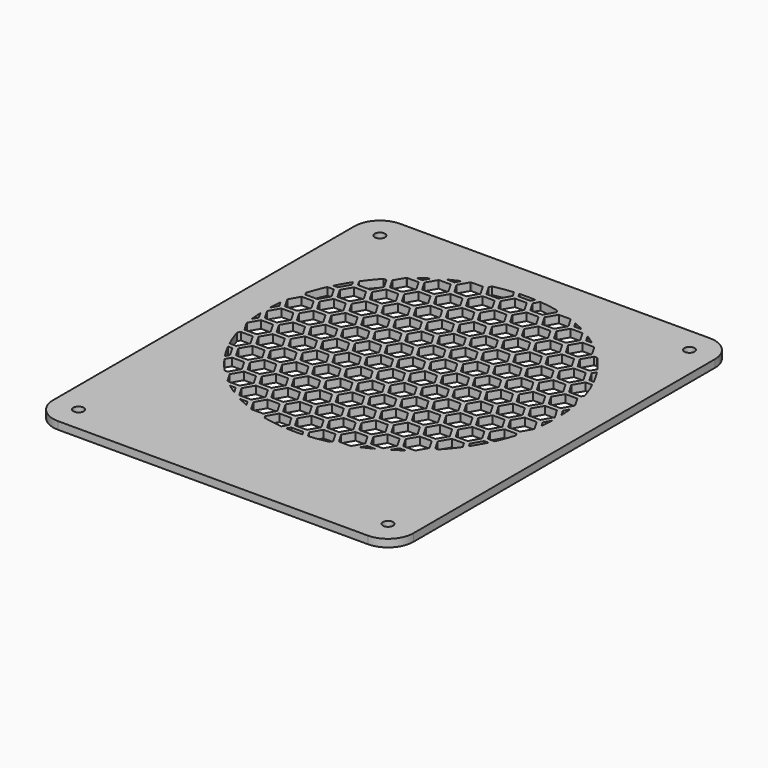
from build123d import *

# Parameters (mm, degrees)
F0_R     = 2
F0_R_2   = 4.5
F1_DEPTH = 3
F2_DEPTH = 2


# Not quite as in the source:
# - ends of sketch curves that miss each other by under 0.0002 mm in the source are joined


with BuildPart() as f1:
    # F0 (on Top) → F1 (new body)
    with BuildSketch(Plane.XY):
        with BuildLine():
            Line((61, 71), (-61, 71))
            ThreePointArc((-61, 71), (-68.0710678119, 68.0710678119), (-71, 61))
            Line((-71, 61), (-71, -87.5))
            ThreePointArc((-71, -87.5), (-68.0710678119, -94.5710678119), (-61, -97.5))
            Line((-61, -97.5), (61, -97.5))
            ThreePointArc((61, -97.5), (68.0710678119, -94.5710678119), (71, -87.5))
            Line((71, -87.5), (71, 61))
            ThreePointArc((71, 61), (68.0710678119, 68.0710678119), (61, 71))
        make_face()
        with Locations((-61, -87.5)):
            Circle(F0_R, mode=Mode.SUBTRACT)
        with Locations((-52.2617718254, -52.3417506076)):
            Circle(F0_R_2, mode=Mode.SUBTRACT)
        with BuildLine():
            Line((-45.6730132859, -30.9579411415), (-40.9387409983, -30.9579411415))
            Line((-40.9387409983, -30.9579411415), (-38.5716048624, -35.0579411973))
            Line((-38.5716048624, -35.0579411973), (-40.9387411583, -39.1579412804))
            Line((-40.9387411583, -39.1579412804), (-42.1058859861, -39.1579412804))
            ThreePointArc((-42.1058859861, -39.1579412804), (-44.6321134172, -36.2522337507), (-46.9582140117, -33.1839740965))
            Line((-46.9582140117, -33.1839740965), (-45.6730132859, -30.9579411415))
        make_face(mode=Mode.SUBTRACT)
        with BuildLine():
            Line((-49.5989950362, -25.9579412533), (-47.2318589003, -30.057941309))
            Line((-47.2318589003, -30.057941309), (-48.0829899864, -31.5321435042))
            ThreePointArc((-48.0829899864, -31.5321435042), (-49.7732212515, -28.7902144182), (-51.3072634808, -25.9579412533))
            Line((-51.3072634808, -25.9579412533), (-49.5989950362, -25.9579412533))
        make_face(mode=Mode.SUBTRACT)
        Polygon((-40.9387409983, -20.8999998188), (-38.5716048624, -24.9999998745), (-40.9387411583, -29.0999999577), (-45.6730132859, -29.0999999577), (-48.0401494297, -24.9999998882), (-45.6730132859, -20.8999998188), align=None, mode=Mode.SUBTRACT)
        with BuildLine():
            Line((-49.5989950362, -15.8999999305), (-47.2318589003, -19.9999999863))
            Line((-47.2318589003, -19.9999999863), (-49.5989951961, -24.1000000695))
            Line((-49.5989951961, -24.1000000695), (-52.205746778, -24.1000000695))
            ThreePointArc((-52.205746778, -24.1000000695), (-53.6933380954, -20.5736589885), (-54.9430464582, -16.9561683729))
            Line((-54.9430464582, -16.9561683729), (-54.3332673237, -15.8999999305))
            Line((-54.3332673237, -15.8999999305), (-49.5989950362, -15.8999999305))
        make_face(mode=Mode.SUBTRACT)
        Polygon((-45.6730132859, -19.0999999577), (-48.0401494297, -14.9999998882), (-45.6730132859, -10.8999998188), (-40.9387409983, -10.8999998188), (-38.5716048624, -14.9999998745), (-40.9387411583, -19.0999999577), align=None, mode=Mode.SUBTRACT)
        with BuildLine():
            Line((-34.5560072312, -45.9579412533), (-32.2738800076, -45.9579412533))
            Line((-32.2738800076, -45.9579412533), (-30.7595285917, -48.5808748462))
            ThreePointArc((-30.7595285917, -48.5808748462), (-32.6840901681, -47.3075073311), (-34.5560072312, -45.9579412533))
        make_face(mode=Mode.SUBTRACT)
        with BuildLine():
            Line((-26.6371586929, -50.9579412533), (-23.6136263521, -50.9579412533))
            Line((-23.6136263521, -50.9579412533), (-22.4784041459, -52.9242037923))
            ThreePointArc((-22.4784041459, -52.9242037923), (-24.5774525803, -51.9826781213), (-26.6371586929, -50.9579412533))
        make_face(mode=Mode.SUBTRACT)
        Polygon((-23.6136263521, -40.9579412533), (-21.2464902162, -45.057941309), (-23.6136265121, -49.1579413922), (-28.3478986397, -49.1579413922), (-30.7150347835, -45.0579413227), (-28.3478986397, -40.9579412533), align=None, mode=Mode.SUBTRACT)
        with BuildLine():
            Line((-39.3752884389, -40.0579413227), (-37.0081522952, -35.9579412533))
            Line((-37.0081522952, -35.9579412533), (-32.2738800076, -35.9579412533))
            Line((-32.2738800076, -35.9579412533), (-29.9067438717, -40.057941309))
            Line((-29.9067438717, -40.057941309), (-32.2738801675, -44.1579413922))
            Line((-32.2738801675, -44.1579413922), (-36.8283343637, -44.1579413922))
            ThreePointArc((-36.8283343637, -44.1579413922), (-37.0033480808, -44.0113875129), (-37.1777786102, -43.8641399963))
            Line((-37.1777786102, -43.8641399963), (-39.3752884389, -40.0579413227))
        make_face(mode=Mode.SUBTRACT)
        Polygon((-30.7150347835, -35.0579413227), (-28.3478986397, -30.9579412533), (-23.6136263521, -30.9579412533), (-21.2464902162, -35.057941309), (-23.6136265121, -39.1579413922), (-28.3478986397, -39.1579413922), align=None, mode=Mode.SUBTRACT)
        with BuildLine():
            Line((-14.9533722834, -45.9579412533), (-12.5862361476, -50.057941309))
            Line((-12.5862361476, -50.057941309), (-14.9533724434, -54.1579413922))
            Line((-14.9533724434, -54.1579413922), (-19.3175408414, -54.1579413922))
            ThreePointArc((-19.3175408414, -54.1579413922), (-19.5515976014, -54.0738849283), (-19.7852886212, -53.9888169363))
            Line((-19.7852886212, -53.9888169363), (-22.0547807148, -50.0579413227))
            Line((-22.0547807148, -50.0579413227), (-19.687644571, -45.9579412533))
            Line((-19.687644571, -45.9579412533), (-14.9533722834, -45.9579412533))
        make_face(mode=Mode.SUBTRACT)
        with BuildLine():
            Line((-6.2931178941, -50.9579412533), (-3.9259817582, -55.057941309))
            Line((-3.9259817582, -55.057941309), (-5.199880045, -57.2643977312))
            ThreePointArc((-5.199880045, -57.2643977312), (-9.030429388, -56.7864538871), (-12.8202778486, -56.0525688607))
            Line((-12.8202778486, -56.0525688607), (-13.3945263254, -55.0579413227))
            Line((-13.3945263254, -55.0579413227), (-11.0273901816, -50.9579412533))
            Line((-11.0273901816, -50.9579412533), (-6.2931178941, -50.9579412533))
        make_face(mode=Mode.SUBTRACT)
        Polygon((-13.3945263254, -45.0579413227), (-11.0273901816, -40.9579412533), (-6.2931178941, -40.9579412533), (-3.9259817582, -45.057941309), (-6.293118054, -49.1579413922), (-11.0273901816, -49.1579413922), align=None, mode=Mode.SUBTRACT)
        Polygon((-19.687644571, -44.1579413922), (-22.0547807148, -40.0579413227), (-19.687644571, -35.9579412533), (-14.9533722834, -35.9579412533), (-12.5862361476, -40.057941309), (-14.9533724434, -44.1579413922), align=None, mode=Mode.SUBTRACT)
        Polygon((-13.3945263254, -35.0579413227), (-11.0273901816, -30.9579412533), (-6.2931178941, -30.9579412533), (-3.9259817582, -35.057941309), (-6.293118054, -39.1579413922), (-11.0273901816, -39.1579413922), align=None, mode=Mode.SUBTRACT)
        Polygon((-32.2738800076, -25.9579412533), (-29.9067438717, -30.057941309), (-32.2738801675, -34.1579413922), (-37.0081522952, -34.1579413922), (-39.3752884389, -30.0579413227), (-37.0081522952, -25.9579412533), align=None, mode=Mode.SUBTRACT)
        Polygon((-21.2464902162, -24.9999999863), (-23.6136265121, -29.1000000695), (-28.3478986397, -29.1000000695), (-30.7150347835, -25), (-28.3478986397, -20.8999999305), (-23.6136263521, -20.8999999305), align=None, mode=Mode.SUBTRACT)
        Polygon((-39.3752884389, -20), (-37.0081522952, -15.8999999305), (-32.2738800076, -15.8999999305), (-29.9067438717, -19.9999999863), (-32.2738801675, -24.1000000695), (-37.0081522952, -24.1000000695), align=None, mode=Mode.SUBTRACT)
        Polygon((-23.6136263521, -10.8999999305), (-21.2464902162, -14.9999999863), (-23.6136265121, -19.1000000695), (-28.3478986397, -19.1000000695), (-30.7150347835, -15), (-28.3478986397, -10.8999999305), align=None, mode=Mode.SUBTRACT)
        Polygon((-22.0547807148, -30.0579413227), (-19.687644571, -25.9579412533), (-14.9533722834, -25.9579412533), (-12.5862361476, -30.057941309), (-14.9533724434, -34.1579413922), (-19.687644571, -34.1579413922), align=None, mode=Mode.SUBTRACT)
        Polygon((-3.9259817582, -24.9999999863), (-6.293118054, -29.1000000695), (-11.0273901816, -29.1000000695), (-13.3945263254, -25), (-11.0273901816, -20.8999999305), (-6.2931178941, -20.8999999305), align=None, mode=Mode.SUBTRACT)
        Polygon((-14.9533722834, -15.8999999305), (-12.5862361476, -19.9999999863), (-14.9533724434, -24.1000000695), (-19.687644571, -24.1000000695), (-22.0547807148, -20), (-19.687644571, -15.8999999305), align=None, mode=Mode.SUBTRACT)
        Polygon((-3.9259817582, -14.9999999863), (-6.293118054, -19.1000000695), (-11.0273901816, -19.1000000695), (-13.3945263254, -15), (-11.0273901816, -10.8999999305), (-6.2931178941, -10.8999999305), align=None, mode=Mode.SUBTRACT)
        with BuildLine():
            Line((-2.3671363196, -55.9579410298), (0, -55.9579410298))
            Line((0, -55.9579410298), (2.3671363196, -55.9579410298))
            Line((2.3671363196, -55.9579410298), (3.2058082538, -57.4105634308))
            ThreePointArc((3.2058082538, -57.4105634308), (0, -57.5), (-3.2058082538, -57.4105634308))
            Line((-3.2058082538, -57.4105634308), (-2.3671363196, -55.9579410298))
        make_face(mode=Mode.SUBTRACT)
        with Locations((61, -87.5)):
            Circle(F0_R, mode=Mode.SUBTRACT)
        with BuildLine():
            Line((5.199880045, -57.2643977312), (3.9259817582, -55.057941309))
            Line((3.9259817582, -55.057941309), (6.2931178941, -50.9579412533))
            Line((6.2931178941, -50.9579412533), (11.0273901816, -50.9579412533))
            Line((11.0273901816, -50.9579412533), (13.3945263254, -55.0579413227))
            Line((13.3945263254, -55.0579413227), (12.8202778486, -56.0525688607))
            ThreePointArc((12.8202778486, -56.0525688607), (9.030429388, -56.7864538871), (5.199880045, -57.2643977312))
        make_face(mode=Mode.SUBTRACT)
        Polygon((-2.3671363196, -45.9579410298), (0, -45.9579410298), (2.3671363196, -45.9579410298), (4.7342724633, -50.0579410992), (2.3671363196, -54.1579411687), (0, -54.1579411687), (-2.3671363196, -54.1579411687), (-4.7342724633, -50.0579410992), align=None, mode=Mode.SUBTRACT)
        Polygon((11.0273901816, -40.9579412533), (13.3945263254, -45.0579413227), (11.0273901816, -49.1579413922), (6.293118054, -49.1579413922), (3.9259817582, -45.057941309), (6.2931178941, -40.9579412533), align=None, mode=Mode.SUBTRACT)
        with BuildLine():
            Line((19.3175408414, -54.1579413922), (14.9533724434, -54.1579413922))
            Line((14.9533724434, -54.1579413922), (12.5862361476, -50.057941309))
            Line((12.5862361476, -50.057941309), (14.9533722834, -45.9579412533))
            Line((14.9533722834, -45.9579412533), (19.687644571, -45.9579412533))
            Line((19.687644571, -45.9579412533), (22.0547807148, -50.0579413227))
            Line((22.0547807148, -50.0579413227), (19.7852886212, -53.9888169363))
            ThreePointArc((19.7852886212, -53.9888169363), (19.5515976014, -54.0738849283), (19.3175408414, -54.1579413922))
        make_face(mode=Mode.SUBTRACT)
        Polygon((2.3671363196, -44.1579411687), (0, -44.1579411687), (-2.3671363196, -44.1579411687), (-4.7342724633, -40.0579410992), (-2.3671363196, -35.9579410298), (0, -35.9579410298), (2.3671363196, -35.9579410298), (4.7342724633, -40.0579410992), align=None, mode=Mode.SUBTRACT)
        Polygon((11.0273901816, -30.9579412533), (13.3945263254, -35.0579413227), (11.0273901816, -39.1579413922), (6.293118054, -39.1579413922), (3.9259817582, -35.057941309), (6.2931178941, -30.9579412533), align=None, mode=Mode.SUBTRACT)
        Polygon((19.687644571, -44.1579413922), (14.9533724434, -44.1579413922), (12.5862361476, -40.057941309), (14.9533722834, -35.9579412533), (19.687644571, -35.9579412533), (22.0547807148, -40.0579413227), align=None, mode=Mode.SUBTRACT)
        with BuildLine():
            ThreePointArc((26.6371586929, -50.9579412533), (24.5774525803, -51.9826781213), (22.4784041459, -52.9242037923))
            Line((22.4784041459, -52.9242037923), (23.6136263521, -50.9579412533))
            Line((23.6136263521, -50.9579412533), (26.6371586929, -50.9579412533))
        make_face(mode=Mode.SUBTRACT)
        Polygon((28.3478986397, -40.9579412533), (30.7150347835, -45.0579413227), (28.3478986397, -49.1579413922), (23.6136265121, -49.1579413922), (21.2464902162, -45.057941309), (23.6136263521, -40.9579412533), align=None, mode=Mode.SUBTRACT)
        with BuildLine():
            ThreePointArc((34.5560072312, -45.9579412533), (32.6840901681, -47.3075073311), (30.7595285917, -48.5808748462))
            Line((30.7595285917, -48.5808748462), (32.2738800076, -45.9579412533))
            Line((32.2738800076, -45.9579412533), (34.5560072312, -45.9579412533))
        make_face(mode=Mode.SUBTRACT)
        Polygon((28.3478986397, -30.9579412533), (30.7150347835, -35.0579413227), (28.3478986397, -39.1579413922), (23.6136265121, -39.1579413922), (21.2464902162, -35.057941309), (23.6136263521, -30.9579412533), align=None, mode=Mode.SUBTRACT)
        with BuildLine():
            Line((32.2738801675, -44.1579413922), (29.9067438717, -40.057941309))
            Line((29.9067438717, -40.057941309), (32.2738800076, -35.9579412533))
            Line((32.2738800076, -35.9579412533), (37.0081522952, -35.9579412533))
            Line((37.0081522952, -35.9579412533), (39.3752884389, -40.0579413227))
            Line((39.3752884389, -40.0579413227), (37.1777786102, -43.8641399963))
            ThreePointArc((37.1777786102, -43.8641399963), (37.0033480808, -44.0113875129), (36.8283343637, -44.1579413922))
            Line((36.8283343637, -44.1579413922), (32.2738801675, -44.1579413922))
        make_face(mode=Mode.SUBTRACT)
        Polygon((-2.3671363196, -25.899999707), (0, -25.899999707), (2.3671363196, -25.899999707), (4.7342724633, -29.9999997765), (2.3671363196, -34.0999998459), (0, -34.0999998459), (-2.3671363196, -34.0999998459), (-4.7342724633, -29.9999997765), align=None, mode=Mode.SUBTRACT)
        Polygon((3.9259817582, -24.9999999863), (6.2931178941, -20.8999999305), (11.0273901816, -20.8999999305), (13.3945263254, -25), (11.0273901816, -29.1000000695), (6.293118054, -29.1000000695), align=None, mode=Mode.SUBTRACT)
        Polygon((14.9533724434, -34.1579413922), (12.5862361476, -30.057941309), (14.9533722834, -25.9579412533), (19.687644571, -25.9579412533), (22.0547807148, -30.0579413227), (19.687644571, -34.1579413922), align=None, mode=Mode.SUBTRACT)
        Polygon((-2.3671363196, -15.899999707), (0, -15.899999707), (2.3671363196, -15.899999707), (4.7342724633, -19.9999997765), (2.3671363196, -24.0999998459), (0, -24.0999998459), (-2.3671363196, -24.0999998459), (-4.7342724633, -19.9999997765), align=None, mode=Mode.SUBTRACT)
        Polygon((6.2931178941, -10.8999999305), (11.0273901816, -10.8999999305), (13.3945263254, -15), (11.0273901816, -19.1000000695), (6.293118054, -19.1000000695), (3.9259817582, -14.9999999863), align=None, mode=Mode.SUBTRACT)
        Polygon((14.9533724434, -24.1000000695), (12.5862361476, -19.9999999863), (14.9533722834, -15.8999999305), (19.687644571, -15.8999999305), (22.0547807148, -20), (19.687644571, -24.1000000695), align=None, mode=Mode.SUBTRACT)
        Polygon((28.3478986397, -29.1000000695), (23.6136265121, -29.1000000695), (21.2464902162, -24.9999999863), (23.6136263521, -20.8999999305), (28.3478986397, -20.8999999305), (30.7150347835, -25), align=None, mode=Mode.SUBTRACT)
        Polygon((37.0081522952, -34.1579413922), (32.2738801675, -34.1579413922), (29.9067438717, -30.057941309), (32.2738800076, -25.9579412533), (37.0081522952, -25.9579412533), (39.3752884389, -30.0579413227), align=None, mode=Mode.SUBTRACT)
        Polygon((23.6136265121, -19.1000000695), (21.2464902162, -14.9999999863), (23.6136263521, -10.8999999305), (28.3478986397, -10.8999999305), (30.7150347835, -15), (28.3478986397, -19.1000000695), align=None, mode=Mode.SUBTRACT)
        Polygon((37.0081522952, -15.8999999305), (39.3752884389, -20), (37.0081522952, -24.1000000695), (32.2738801675, -24.1000000695), (29.9067438717, -19.9999999863), (32.2738800076, -15.8999999305), align=None, mode=Mode.SUBTRACT)
        with Locations((52.7382281746, -52.3417506076)):
            Circle(F0_R_2, mode=Mode.SUBTRACT)
        with BuildLine():
            Line((38.5716048624, -35.0579411973), (40.9387409983, -30.9579411415))
            Line((40.9387409983, -30.9579411415), (45.6730132859, -30.9579411415))
            Line((45.6730132859, -30.9579411415), (46.9582140117, -33.1839740965))
            ThreePointArc((46.9582140117, -33.1839740965), (44.6321134172, -36.2522337507), (42.1058859861, -39.1579412804))
            Line((42.1058859861, -39.1579412804), (40.9387411583, -39.1579412804))
            Line((40.9387411583, -39.1579412804), (38.5716048624, -35.0579411973))
        make_face(mode=Mode.SUBTRACT)
        Polygon((38.5716048624, -24.9999998745), (40.9387409983, -20.8999998188), (45.6730132859, -20.8999998188), (48.0401494297, -24.9999998882), (45.6730132859, -29.0999999577), (40.9387411583, -29.0999999577), align=None, mode=Mode.SUBTRACT)
        with BuildLine():
            Line((47.2318589003, -30.057941309), (49.5989950362, -25.9579412533))
            Line((49.5989950362, -25.9579412533), (51.3072634808, -25.9579412533))
            ThreePointArc((51.3072634808, -25.9579412533), (49.7732212515, -28.7902144182), (48.0829899864, -31.5321435042))
            Line((48.0829899864, -31.5321435042), (47.2318589003, -30.057941309))
        make_face(mode=Mode.SUBTRACT)
        Polygon((45.6730132859, -10.8999998188), (48.0401494297, -14.9999998882), (45.6730132859, -19.0999999577), (40.9387411583, -19.0999999577), (38.5716048624, -14.9999998745), (40.9387409983, -10.8999998188), align=None, mode=Mode.SUBTRACT)
        with BuildLine():
            Line((49.5989951961, -24.1000000695), (47.2318589003, -19.9999999863))
            Line((47.2318589003, -19.9999999863), (49.5989950362, -15.8999999305))
            Line((49.5989950362, -15.8999999305), (54.3332673237, -15.8999999305))
            Line((54.3332673237, -15.8999999305), (54.9430464582, -16.9561683729))
            ThreePointArc((54.9430464582, -16.9561683729), (53.6933380954, -20.5736589885), (52.205746778, -24.1000000695))
            Line((52.205746778, -24.1000000695), (49.5989951961, -24.1000000695))
        make_face(mode=Mode.SUBTRACT)
        with BuildLine():
            Line((-57.4538634934, -2.3029480405), (-55.896719891, -4.9999998745))
            Line((-55.896719891, -4.9999998745), (-57.0686536481, -7.0298485613))
            ThreePointArc((-57.0686536481, -7.0298485613), (-57.3100133506, -4.6703714797), (-57.4538634934, -2.3029480405))
        make_face(mode=Mode.SUBTRACT)
        with BuildLine():
            Line((-57.0686536481, 7.0298485613), (-55.896719891, 4.9999998745))
            Line((-55.896719891, 4.9999998745), (-57.4538634934, 2.3029480405))
            ThreePointArc((-57.4538634934, 2.3029480405), (-57.3100133506, 4.6703714797), (-57.0686536481, 7.0298485613))
        make_face(mode=Mode.SUBTRACT)
        with BuildLine():
            Line((-54.3332673237, -5.8999999305), (-49.5989950362, -5.8999999305))
            Line((-49.5989950362, -5.8999999305), (-47.2318589003, -9.9999999863))
            Line((-47.2318589003, -9.9999999863), (-49.5989951961, -14.1000000695))
            Line((-49.5989951961, -14.1000000695), (-54.3332673237, -14.1000000695))
            Line((-54.3332673237, -14.1000000695), (-56.5894972032, -10.1920952847))
            ThreePointArc((-56.5894972032, -10.1920952847), (-56.6157588926, -10.0451901433), (-56.6416392201, -9.8982173377))
            Line((-56.6416392201, -9.8982173377), (-54.3332673237, -5.8999999305))
        make_face(mode=Mode.SUBTRACT)
        Polygon((-48.0401494297, -4.9999998882), (-45.6730132859, -0.8999998188), (-40.9387409983, -0.8999998188), (-38.5716048624, -4.9999998745), (-40.9387411583, -9.0999999577), (-45.6730132859, -9.0999999577), align=None, mode=Mode.SUBTRACT)
        Polygon((-54.3332673237, 4.1000000695), (-49.5989951961, 4.1000000695), (-47.2318589003, -1.37e-08), (-49.5989951961, -4.1000000695), (-54.3332673237, -4.1000000695), (-56.7004034675, 0), align=None, mode=Mode.SUBTRACT)
        Polygon((-38.5716048624, 4.9999998745), (-40.9387409983, 0.8999998188), (-45.6730132859, 0.8999998188), (-48.0401494297, 4.9999998882), (-45.6730132859, 9.0999999577), (-40.9387411583, 9.0999999577), align=None, mode=Mode.SUBTRACT)
        with BuildLine():
            ThreePointArc((-56.6416392201, 9.8982173377), (-56.6157588926, 10.0451901433), (-56.5894972032, 10.1920952847))
            Line((-56.5894972032, 10.1920952847), (-54.3332673237, 14.1000000695))
            Line((-54.3332673237, 14.1000000695), (-49.5989951961, 14.1000000695))
            Line((-49.5989951961, 14.1000000695), (-47.2318589003, 9.9999999863))
            Line((-47.2318589003, 9.9999999863), (-49.5989950362, 5.8999999305))
            Line((-49.5989950362, 5.8999999305), (-54.3332673237, 5.8999999305))
            Line((-54.3332673237, 5.8999999305), (-56.6416392201, 9.8982173377))
        make_face(mode=Mode.SUBTRACT)
        Polygon((-40.9387411583, 19.0999999577), (-38.5716048624, 14.9999998745), (-40.9387409983, 10.8999998188), (-45.6730132859, 10.8999998188), (-48.0401494297, 14.9999998882), (-45.6730132859, 19.0999999577), align=None, mode=Mode.SUBTRACT)
        with BuildLine():
            Line((-47.2318589003, 19.9999999863), (-49.5989950362, 15.8999999305))
            Line((-49.5989950362, 15.8999999305), (-54.3332673237, 15.8999999305))
            Line((-54.3332673237, 15.8999999305), (-54.9430464582, 16.9561683729))
            ThreePointArc((-54.9430464582, 16.9561683729), (-53.6933380954, 20.5736589885), (-52.205746778, 24.1000000695))
            Line((-52.205746778, 24.1000000695), (-49.5989951961, 24.1000000695))
            Line((-49.5989951961, 24.1000000695), (-47.2318589003, 19.9999999863))
        make_face(mode=Mode.SUBTRACT)
        with BuildLine():
            Line((-48.0829899864, 31.5321435042), (-47.2318589003, 30.057941309))
            Line((-47.2318589003, 30.057941309), (-49.5989950362, 25.9579412533))
            Line((-49.5989950362, 25.9579412533), (-51.3072634808, 25.9579412533))
            ThreePointArc((-51.3072634808, 25.9579412533), (-49.7732212515, 28.7902144182), (-48.0829899864, 31.5321435042))
        make_face(mode=Mode.SUBTRACT)
        Polygon((-45.6730132859, 29.0999999577), (-40.9387411583, 29.0999999577), (-38.5716048624, 24.9999998745), (-40.9387409983, 20.8999998188), (-45.6730132859, 20.8999998188), (-48.0401494297, 24.9999998882), align=None, mode=Mode.SUBTRACT)
        Polygon((-37.0081522952, -14.1000000695), (-39.3752884389, -10), (-37.0081522952, -5.8999999305), (-32.2738800076, -5.8999999305), (-29.9067438717, -9.9999999863), (-32.2738801675, -14.1000000695), align=None, mode=Mode.SUBTRACT)
        Polygon((-30.7150347835, -5), (-28.3478986397, -0.8999999305), (-23.6136263521, -0.8999999305), (-21.2464902162, -4.9999999863), (-23.6136265121, -9.1000000695), (-28.3478986397, -9.1000000695), align=None, mode=Mode.SUBTRACT)
        Polygon((-32.2738801675, 4.1000000695), (-29.9067438717, -1.37e-08), (-32.2738801675, -4.1000000695), (-37.0081522952, -4.1000000695), (-39.3752884389, 0), (-37.0081522952, 4.1000000695), align=None, mode=Mode.SUBTRACT)
        Polygon((-28.3478986397, 0.8999999305), (-30.7150347835, 5), (-28.3478986397, 9.1000000695), (-23.6136265121, 9.1000000695), (-21.2464902162, 4.9999999863), (-23.6136263521, 0.8999999305), align=None, mode=Mode.SUBTRACT)
        Polygon((-19.687644571, -5.8999999305), (-14.9533722834, -5.8999999305), (-12.5862361476, -9.9999999863), (-14.9533724434, -14.1000000695), (-19.687644571, -14.1000000695), (-22.0547807148, -10), align=None, mode=Mode.SUBTRACT)
        Polygon((-13.3945263254, -5), (-11.0273901816, -0.8999999305), (-6.2931178941, -0.8999999305), (-3.9259817582, -4.9999999863), (-6.293118054, -9.1000000695), (-11.0273901816, -9.1000000695), align=None, mode=Mode.SUBTRACT)
        Polygon((-19.687644571, -4.1000000695), (-22.0547807148, 0), (-19.687644571, 4.1000000695), (-14.9533724434, 4.1000000695), (-12.5862361476, -1.37e-08), (-14.9533724434, -4.1000000695), align=None, mode=Mode.SUBTRACT)
        Polygon((-11.0273901816, 9.1000000695), (-6.293118054, 9.1000000695), (-3.9259817582, 4.9999999863), (-6.2931178941, 0.8999999305), (-11.0273901816, 0.8999999305), (-13.3945263254, 5), align=None, mode=Mode.SUBTRACT)
        Polygon((-32.2738801675, 14.1000000695), (-29.9067438717, 9.9999999863), (-32.2738800076, 5.8999999305), (-37.0081522952, 5.8999999305), (-39.3752884389, 10), (-37.0081522952, 14.1000000695), align=None, mode=Mode.SUBTRACT)
        Polygon((-23.6136265121, 19.1000000695), (-21.2464902162, 14.9999999863), (-23.6136263521, 10.8999999305), (-28.3478986397, 10.8999999305), (-30.7150347835, 15), (-28.3478986397, 19.1000000695), align=None, mode=Mode.SUBTRACT)
        Polygon((-32.2738801675, 24.1000000695), (-29.9067438717, 19.9999999863), (-32.2738800076, 15.8999999305), (-37.0081522952, 15.8999999305), (-39.3752884389, 20), (-37.0081522952, 24.1000000695), align=None, mode=Mode.SUBTRACT)
        Polygon((-23.6136263521, 20.8999999305), (-28.3478986397, 20.8999999305), (-30.7150347835, 25), (-28.3478986397, 29.1000000695), (-23.6136265121, 29.1000000695), (-21.2464902162, 24.9999999863), align=None, mode=Mode.SUBTRACT)
        Polygon((-12.5862361476, 9.9999999863), (-14.9533722834, 5.8999999305), (-19.687644571, 5.8999999305), (-22.0547807148, 10), (-19.687644571, 14.1000000695), (-14.9533724434, 14.1000000695), align=None, mode=Mode.SUBTRACT)
        Polygon((-11.0273901816, 19.1000000695), (-6.293118054, 19.1000000695), (-3.9259817582, 14.9999999863), (-6.2931178941, 10.8999999305), (-11.0273901816, 10.8999999305), (-13.3945263254, 15), align=None, mode=Mode.SUBTRACT)
        Polygon((-19.687644571, 15.8999999305), (-22.0547807148, 20), (-19.687644571, 24.1000000695), (-14.9533724434, 24.1000000695), (-12.5862361476, 19.9999999863), (-14.9533722834, 15.8999999305), align=None, mode=Mode.SUBTRACT)
        Polygon((-11.0273901816, 20.8999999305), (-13.3945263254, 25), (-11.0273901816, 29.1000000695), (-6.293118054, 29.1000000695), (-3.9259817582, 24.9999999863), (-6.2931178941, 20.8999999305), align=None, mode=Mode.SUBTRACT)
        with BuildLine():
            Line((-40.9387409983, 30.9579411415), (-45.6730132859, 30.9579411415))
            Line((-45.6730132859, 30.9579411415), (-46.9582140117, 33.1839740965))
            ThreePointArc((-46.9582140117, 33.1839740965), (-44.6321134172, 36.2522337507), (-42.1058859861, 39.1579412804))
            Line((-42.1058859861, 39.1579412804), (-40.9387411583, 39.1579412804))
            Line((-40.9387411583, 39.1579412804), (-38.5716048624, 35.0579411973))
            Line((-38.5716048624, 35.0579411973), (-40.9387409983, 30.9579411415))
        make_face(mode=Mode.SUBTRACT)
        with Locations((-61, 61)):
            Circle(F0_R, mode=Mode.SUBTRACT)
        with Locations((-52.5, 52.5)):
            Circle(F0_R_2, mode=Mode.SUBTRACT)
        Polygon((-37.0081522952, 34.1579413922), (-32.2738801675, 34.1579413922), (-29.9067438717, 30.057941309), (-32.2738800076, 25.9579412533), (-37.0081522952, 25.9579412533), (-39.3752884389, 30.0579413227), align=None, mode=Mode.SUBTRACT)
        Polygon((-21.2464902162, 35.057941309), (-23.6136263521, 30.9579412533), (-28.3478986397, 30.9579412533), (-30.7150347835, 35.0579413227), (-28.3478986397, 39.1579413922), (-23.6136265121, 39.1579413922), align=None, mode=Mode.SUBTRACT)
        with BuildLine():
            Line((-32.2738801675, 44.1579413922), (-29.9067438717, 40.057941309))
            Line((-29.9067438717, 40.057941309), (-32.2738800076, 35.9579412533))
            Line((-32.2738800076, 35.9579412533), (-37.0081522952, 35.9579412533))
            Line((-37.0081522952, 35.9579412533), (-39.3752884389, 40.0579413227))
            Line((-39.3752884389, 40.0579413227), (-37.1777786102, 43.8641399963))
            ThreePointArc((-37.1777786102, 43.8641399963), (-37.0033480808, 44.0113875129), (-36.8283343637, 44.1579413922))
            Line((-36.8283343637, 44.1579413922), (-32.2738801675, 44.1579413922))
        make_face(mode=Mode.SUBTRACT)
        with BuildLine():
            Line((-30.7595285917, 48.5808748462), (-32.2738800076, 45.9579412533))
            Line((-32.2738800076, 45.9579412533), (-34.5560072312, 45.9579412533))
            ThreePointArc((-34.5560072312, 45.9579412533), (-32.6840901681, 47.3075073311), (-30.7595285917, 48.5808748462))
        make_face(mode=Mode.SUBTRACT)
        Polygon((-23.6136265121, 49.1579413922), (-21.2464902162, 45.057941309), (-23.6136263521, 40.9579412533), (-28.3478986397, 40.9579412533), (-30.7150347835, 45.0579413227), (-28.3478986397, 49.1579413922), align=None, mode=Mode.SUBTRACT)
        Polygon((-19.687644571, 34.1579413922), (-14.9533724434, 34.1579413922), (-12.5862361476, 30.057941309), (-14.9533722834, 25.9579412533), (-19.687644571, 25.9579412533), (-22.0547807148, 30.0579413227), align=None, mode=Mode.SUBTRACT)
        Polygon((-6.293118054, 39.1579413922), (-3.9259817582, 35.057941309), (-6.2931178941, 30.9579412533), (-11.0273901816, 30.9579412533), (-13.3945263254, 35.0579413227), (-11.0273901816, 39.1579413922), align=None, mode=Mode.SUBTRACT)
        Polygon((-12.5862361476, 40.057941309), (-14.9533722834, 35.9579412533), (-19.687644571, 35.9579412533), (-22.0547807148, 40.0579413227), (-19.687644571, 44.1579413922), (-14.9533724434, 44.1579413922), align=None, mode=Mode.SUBTRACT)
        Polygon((-6.293118054, 49.1579413922), (-3.9259817582, 45.057941309), (-6.2931178941, 40.9579412533), (-11.0273901816, 40.9579412533), (-13.3945263254, 45.0579413227), (-11.0273901816, 49.1579413922), align=None, mode=Mode.SUBTRACT)
        with BuildLine():
            Line((-22.4784041459, 52.9242037923), (-23.6136263521, 50.9579412533))
            Line((-23.6136263521, 50.9579412533), (-26.6371586929, 50.9579412533))
            ThreePointArc((-26.6371586929, 50.9579412533), (-24.5774525803, 51.9826781213), (-22.4784041459, 52.9242037923))
        make_face(mode=Mode.SUBTRACT)
        with BuildLine():
            Line((-19.687644571, 45.9579412533), (-22.0547807148, 50.0579413227))
            Line((-22.0547807148, 50.0579413227), (-19.7852886212, 53.9888169363))
            ThreePointArc((-19.7852886212, 53.9888169363), (-19.5515976014, 54.0738849283), (-19.3175408414, 54.1579413922))
            Line((-19.3175408414, 54.1579413922), (-14.9533724434, 54.1579413922))
            Line((-14.9533724434, 54.1579413922), (-12.5862361476, 50.057941309))
            Line((-12.5862361476, 50.057941309), (-14.9533722834, 45.9579412533))
            Line((-14.9533722834, 45.9579412533), (-19.687644571, 45.9579412533))
        make_face(mode=Mode.SUBTRACT)
        with BuildLine():
            Line((-6.2931178941, 50.9579412533), (-11.0273901816, 50.9579412533))
            Line((-11.0273901816, 50.9579412533), (-13.3945263254, 55.0579413227))
            Line((-13.3945263254, 55.0579413227), (-12.8202778486, 56.0525688607))
            ThreePointArc((-12.8202778486, 56.0525688607), (-9.030429388, 56.7864538871), (-5.199880045, 57.2643977312))
            Line((-5.199880045, 57.2643977312), (-3.9259817582, 55.057941309))
            Line((-3.9259817582, 55.057941309), (-6.2931178941, 50.9579412533))
        make_face(mode=Mode.SUBTRACT)
        Polygon((2.3671363196, -14.0999998459), (0, -14.0999998459), (-2.3671363196, -14.0999998459), (-4.7342724633, -9.9999997765), (-2.3671363196, -5.899999707), (0, -5.899999707), (2.3671363196, -5.899999707), (4.7342724633, -9.9999997765), align=None, mode=Mode.SUBTRACT)
        Polygon((6.293118054, -9.1000000695), (3.9259817582, -4.9999999863), (6.2931178941, -0.8999999305), (11.0273901816, -0.8999999305), (13.3945263254, -5), (11.0273901816, -9.1000000695), align=None, mode=Mode.SUBTRACT)
        Polygon((19.687644571, -5.8999999305), (22.0547807148, -10), (19.687644571, -14.1000000695), (14.9533724434, -14.1000000695), (12.5862361476, -9.9999999863), (14.9533722834, -5.8999999305), align=None, mode=Mode.SUBTRACT)
        Polygon((-2.367135968, 4.0999999577), (0, 4.0999999577), (2.367135968, 4.0999999577), (4.7342721118, -1.118e-07), (2.367135968, -4.0999999577), (0, -4.0999999577), (-2.367135968, -4.0999999577), (-4.7342721118, 1.118e-07), align=None, mode=Mode.SUBTRACT)
        Polygon((6.2931178941, 0.8999999305), (3.9259817582, 4.9999999863), (6.293118054, 9.1000000695), (11.0273901816, 9.1000000695), (13.3945263254, 5), (11.0273901816, 0.8999999305), align=None, mode=Mode.SUBTRACT)
        Polygon((12.5862361476, -1.37e-08), (14.9533724434, 4.1000000695), (19.687644571, 4.1000000695), (22.0547807148, 0), (19.687644571, -4.1000000695), (14.9533724434, -4.1000000695), align=None, mode=Mode.SUBTRACT)
        Polygon((23.6136263521, -0.8999999305), (28.3478986397, -0.8999999305), (30.7150347835, -5), (28.3478986397, -9.1000000695), (23.6136265121, -9.1000000695), (21.2464902162, -4.9999999863), align=None, mode=Mode.SUBTRACT)
        Polygon((32.2738801675, -14.1000000695), (29.9067438717, -9.9999999863), (32.2738800076, -5.8999999305), (37.0081522952, -5.8999999305), (39.3752884389, -10), (37.0081522952, -14.1000000695), align=None, mode=Mode.SUBTRACT)
        Polygon((23.6136263521, 0.8999999305), (21.2464902162, 4.9999999863), (23.6136265121, 9.1000000695), (28.3478986397, 9.1000000695), (30.7150347835, 5), (28.3478986397, 0.8999999305), align=None, mode=Mode.SUBTRACT)
        Polygon((29.9067438717, -1.37e-08), (32.2738801675, 4.1000000695), (37.0081522952, 4.1000000695), (39.3752884389, 0), (37.0081522952, -4.1000000695), (32.2738801675, -4.1000000695), align=None, mode=Mode.SUBTRACT)
        Polygon((-2.3671363196, 14.0999998459), (0, 14.0999998459), (2.3671363196, 14.0999998459), (4.7342724633, 9.9999997765), (2.3671363196, 5.899999707), (0, 5.899999707), (-2.3671363196, 5.899999707), (-4.7342724633, 9.9999997765), align=None, mode=Mode.SUBTRACT)
        Polygon((6.2931178941, 10.8999999305), (3.9259817582, 14.9999999863), (6.293118054, 19.1000000695), (11.0273901816, 19.1000000695), (13.3945263254, 15), (11.0273901816, 10.8999999305), align=None, mode=Mode.SUBTRACT)
        Polygon((14.9533722834, 5.8999999305), (12.5862361476, 9.9999999863), (14.9533724434, 14.1000000695), (19.687644571, 14.1000000695), (22.0547807148, 10), (19.687644571, 5.8999999305), align=None, mode=Mode.SUBTRACT)
        Polygon((-2.3671363196, 24.0999998459), (0, 24.0999998459), (2.3671363196, 24.0999998459), (4.7342724633, 19.9999997765), (2.3671363196, 15.899999707), (0, 15.899999707), (-2.3671363196, 15.899999707), (-4.7342724633, 19.9999997765), align=None, mode=Mode.SUBTRACT)
        Polygon((6.2931178941, 20.8999999305), (3.9259817582, 24.9999999863), (6.293118054, 29.1000000695), (11.0273901816, 29.1000000695), (13.3945263254, 25), (11.0273901816, 20.8999999305), align=None, mode=Mode.SUBTRACT)
        Polygon((14.9533722834, 15.8999999305), (12.5862361476, 19.9999999863), (14.9533724434, 24.1000000695), (19.687644571, 24.1000000695), (22.0547807148, 20), (19.687644571, 15.8999999305), align=None, mode=Mode.SUBTRACT)
        Polygon((23.6136263521, 10.8999999305), (21.2464902162, 14.9999999863), (23.6136265121, 19.1000000695), (28.3478986397, 19.1000000695), (30.7150347835, 15), (28.3478986397, 10.8999999305), align=None, mode=Mode.SUBTRACT)
        Polygon((32.2738800076, 5.8999999305), (29.9067438717, 9.9999999863), (32.2738801675, 14.1000000695), (37.0081522952, 14.1000000695), (39.3752884389, 10), (37.0081522952, 5.8999999305), align=None, mode=Mode.SUBTRACT)
        Polygon((23.6136263521, 20.8999999305), (21.2464902162, 24.9999999863), (23.6136265121, 29.1000000695), (28.3478986397, 29.1000000695), (30.7150347835, 25), (28.3478986397, 20.8999999305), align=None, mode=Mode.SUBTRACT)
        Polygon((32.2738800076, 15.8999999305), (29.9067438717, 19.9999999863), (32.2738801675, 24.1000000695), (37.0081522952, 24.1000000695), (39.3752884389, 20), (37.0081522952, 15.8999999305), align=None, mode=Mode.SUBTRACT)
        Polygon((45.6730132859, -9.0999999577), (40.9387411583, -9.0999999577), (38.5716048624, -4.9999998745), (40.9387409983, -0.8999998188), (45.6730132859, -0.8999998188), (48.0401494297, -4.9999998882), align=None, mode=Mode.SUBTRACT)
        with BuildLine():
            ThreePointArc((56.6416392201, -9.8982173377), (56.6157588926, -10.0451901433), (56.5894972032, -10.1920952847))
            Line((56.5894972032, -10.1920952847), (54.3332673237, -14.1000000695))
            Line((54.3332673237, -14.1000000695), (49.5989951961, -14.1000000695))
            Line((49.5989951961, -14.1000000695), (47.2318589003, -9.9999999863))
            Line((47.2318589003, -9.9999999863), (49.5989950362, -5.8999999305))
            Line((49.5989950362, -5.8999999305), (54.3332673237, -5.8999999305))
            Line((54.3332673237, -5.8999999305), (56.6416392201, -9.8982173377))
        make_face(mode=Mode.SUBTRACT)
        Polygon((40.9387409983, 0.8999998188), (38.5716048624, 4.9999998745), (40.9387411583, 9.0999999577), (45.6730132859, 9.0999999577), (48.0401494297, 4.9999998882), (45.6730132859, 0.8999998188), align=None, mode=Mode.SUBTRACT)
        Polygon((47.2318589003, -1.37e-08), (49.5989951961, 4.1000000695), (54.3332673237, 4.1000000695), (56.7004034675, 0), (54.3332673237, -4.1000000695), (49.5989951961, -4.1000000695), align=None, mode=Mode.SUBTRACT)
        with BuildLine():
            Line((57.0686536481, -7.0298485613), (55.896719891, -4.9999998745))
            Line((55.896719891, -4.9999998745), (57.4538634934, -2.3029480405))
            ThreePointArc((57.4538634934, -2.3029480405), (57.3100133506, -4.6703714797), (57.0686536481, -7.0298485613))
        make_face(mode=Mode.SUBTRACT)
        with BuildLine():
            ThreePointArc((57.0686536481, 7.0298485613), (57.3100133506, 4.6703714797), (57.4538634934, 2.3029480405))
            Line((57.4538634934, 2.3029480405), (55.896719891, 4.9999998745))
            Line((55.896719891, 4.9999998745), (57.0686536481, 7.0298485613))
        make_face(mode=Mode.SUBTRACT)
        Polygon((40.9387409983, 10.8999998188), (38.5716048624, 14.9999998745), (40.9387411583, 19.0999999577), (45.6730132859, 19.0999999577), (48.0401494297, 14.9999998882), (45.6730132859, 10.8999998188), align=None, mode=Mode.SUBTRACT)
        with BuildLine():
            Line((49.5989950362, 5.8999999305), (47.2318589003, 9.9999999863))
            Line((47.2318589003, 9.9999999863), (49.5989951961, 14.1000000695))
            Line((49.5989951961, 14.1000000695), (54.3332673237, 14.1000000695))
            Line((54.3332673237, 14.1000000695), (56.5894972032, 10.1920952847))
            ThreePointArc((56.5894972032, 10.1920952847), (56.6157588926, 10.0451901433), (56.6416392201, 9.8982173377))
            Line((56.6416392201, 9.8982173377), (54.3332673237, 5.8999999305))
            Line((54.3332673237, 5.8999999305), (49.5989950362, 5.8999999305))
        make_face(mode=Mode.SUBTRACT)
        Polygon((40.9387409983, 20.8999998188), (38.5716048624, 24.9999998745), (40.9387411583, 29.0999999577), (45.6730132859, 29.0999999577), (48.0401494297, 24.9999998882), (45.6730132859, 20.8999998188), align=None, mode=Mode.SUBTRACT)
        with BuildLine():
            Line((49.5989950362, 15.8999999305), (47.2318589003, 19.9999999863))
            Line((47.2318589003, 19.9999999863), (49.5989951961, 24.1000000695))
            Line((49.5989951961, 24.1000000695), (52.205746778, 24.1000000695))
            ThreePointArc((52.205746778, 24.1000000695), (53.6933380954, 20.5736589885), (54.9430464582, 16.9561683729))
            Line((54.9430464582, 16.9561683729), (54.3332673237, 15.8999999305))
            Line((54.3332673237, 15.8999999305), (49.5989950362, 15.8999999305))
        make_face(mode=Mode.SUBTRACT)
        with BuildLine():
            Line((49.5989950362, 25.9579412533), (47.2318589003, 30.057941309))
            Line((47.2318589003, 30.057941309), (48.0829899864, 31.5321435042))
            ThreePointArc((48.0829899864, 31.5321435042), (49.7732212515, 28.7902144182), (51.3072634808, 25.9579412533))
            Line((51.3072634808, 25.9579412533), (49.5989950362, 25.9579412533))
        make_face(mode=Mode.SUBTRACT)
        Polygon((-2.3671363196, 34.0999998459), (0, 34.0999998459), (2.3671363196, 34.0999998459), (4.7342724633, 29.9999997765), (2.3671363196, 25.899999707), (0, 25.899999707), (-2.3671363196, 25.899999707), (-4.7342724633, 29.9999997765), align=None, mode=Mode.SUBTRACT)
        Polygon((6.2931178941, 30.9579412533), (3.9259817582, 35.057941309), (6.293118054, 39.1579413922), (11.0273901816, 39.1579413922), (13.3945263254, 35.0579413227), (11.0273901816, 30.9579412533), align=None, mode=Mode.SUBTRACT)
        Polygon((14.9533722834, 25.9579412533), (12.5862361476, 30.057941309), (14.9533724434, 34.1579413922), (19.687644571, 34.1579413922), (22.0547807148, 30.0579413227), (19.687644571, 25.9579412533), align=None, mode=Mode.SUBTRACT)
        Polygon((-2.3671363196, 44.1579411687), (0, 44.1579411687), (2.3671363196, 44.1579411687), (4.7342724633, 40.0579410992), (2.3671363196, 35.9579410298), (0, 35.9579410298), (-2.3671363196, 35.9579410298), (-4.7342724633, 40.0579410992), align=None, mode=Mode.SUBTRACT)
        Polygon((6.2931178941, 40.9579412533), (3.9259817582, 45.057941309), (6.293118054, 49.1579413922), (11.0273901816, 49.1579413922), (13.3945263254, 45.0579413227), (11.0273901816, 40.9579412533), align=None, mode=Mode.SUBTRACT)
        Polygon((14.9533722834, 35.9579412533), (12.5862361476, 40.057941309), (14.9533724434, 44.1579413922), (19.687644571, 44.1579413922), (22.0547807148, 40.0579413227), (19.687644571, 35.9579412533), align=None, mode=Mode.SUBTRACT)
        Polygon((23.6136263521, 30.9579412533), (21.2464902162, 35.057941309), (23.6136265121, 39.1579413922), (28.3478986397, 39.1579413922), (30.7150347835, 35.0579413227), (28.3478986397, 30.9579412533), align=None, mode=Mode.SUBTRACT)
        Polygon((32.2738800076, 25.9579412533), (29.9067438717, 30.057941309), (32.2738801675, 34.1579413922), (37.0081522952, 34.1579413922), (39.3752884389, 30.0579413227), (37.0081522952, 25.9579412533), align=None, mode=Mode.SUBTRACT)
        Polygon((23.6136263521, 40.9579412533), (21.2464902162, 45.057941309), (23.6136265121, 49.1579413922), (28.3478986397, 49.1579413922), (30.7150347835, 45.0579413227), (28.3478986397, 40.9579412533), align=None, mode=Mode.SUBTRACT)
        with BuildLine():
            Line((32.2738800076, 35.9579412533), (29.9067438717, 40.057941309))
            Line((29.9067438717, 40.057941309), (32.2738801675, 44.1579413922))
            Line((32.2738801675, 44.1579413922), (36.8283343637, 44.1579413922))
            ThreePointArc((36.8283343637, 44.1579413922), (37.0033480808, 44.0113875129), (37.1777786102, 43.8641399963))
            Line((37.1777786102, 43.8641399963), (39.3752884389, 40.0579413227))
            Line((39.3752884389, 40.0579413227), (37.0081522952, 35.9579412533))
            Line((37.0081522952, 35.9579412533), (32.2738800076, 35.9579412533))
        make_face(mode=Mode.SUBTRACT)
        with BuildLine():
            Line((32.2738800076, 45.9579412533), (30.7595285917, 48.5808748462))
            ThreePointArc((30.7595285917, 48.5808748462), (32.6840901681, 47.3075073311), (34.5560072312, 45.9579412533))
            Line((34.5560072312, 45.9579412533), (32.2738800076, 45.9579412533))
        make_face(mode=Mode.SUBTRACT)
        Polygon((-2.3671363196, 54.1579411687), (0, 54.1579411687), (2.3671363196, 54.1579411687), (4.7342724633, 50.0579410992), (2.3671363196, 45.9579410298), (0, 45.9579410298), (-2.3671363196, 45.9579410298), (-4.7342724633, 50.0579410992), align=None, mode=Mode.SUBTRACT)
        with BuildLine():
            Line((6.2931178941, 50.9579412533), (3.9259817582, 55.057941309))
            Line((3.9259817582, 55.057941309), (5.199880045, 57.2643977312))
            ThreePointArc((5.199880045, 57.2643977312), (9.030429388, 56.7864538871), (12.8202778486, 56.0525688607))
            Line((12.8202778486, 56.0525688607), (13.3945263254, 55.0579413227))
            Line((13.3945263254, 55.0579413227), (11.0273901816, 50.9579412533))
            Line((11.0273901816, 50.9579412533), (6.2931178941, 50.9579412533))
        make_face(mode=Mode.SUBTRACT)
        with BuildLine():
            Line((0, 55.9579410298), (-2.3671363196, 55.9579410298))
            Line((-2.3671363196, 55.9579410298), (-3.2058082538, 57.4105634308))
            ThreePointArc((-3.2058082538, 57.4105634308), (0, 57.5), (3.2058082538, 57.4105634308))
            Line((3.2058082538, 57.4105634308), (2.3671363196, 55.9579410298))
            Line((2.3671363196, 55.9579410298), (0, 55.9579410298))
        make_face(mode=Mode.SUBTRACT)
        with BuildLine():
            Line((14.9533722834, 45.9579412533), (12.5862361476, 50.057941309))
            Line((12.5862361476, 50.057941309), (14.9533724434, 54.1579413922))
            Line((14.9533724434, 54.1579413922), (19.3175408414, 54.1579413922))
            ThreePointArc((19.3175408414, 54.1579413922), (19.5515976014, 54.0738849283), (19.7852886212, 53.9888169363))
            Line((19.7852886212, 53.9888169363), (22.0547807148, 50.0579413227))
            Line((22.0547807148, 50.0579413227), (19.687644571, 45.9579412533))
            Line((19.687644571, 45.9579412533), (14.9533722834, 45.9579412533))
        make_face(mode=Mode.SUBTRACT)
        with BuildLine():
            Line((23.6136263521, 50.9579412533), (22.4784041459, 52.9242037923))
            ThreePointArc((22.4784041459, 52.9242037923), (24.5774525803, 51.9826781213), (26.6371586929, 50.9579412533))
            Line((26.6371586929, 50.9579412533), (23.6136263521, 50.9579412533))
        make_face(mode=Mode.SUBTRACT)
        with BuildLine():
            Line((40.9387409983, 30.9579411415), (38.5716048624, 35.0579411973))
            Line((38.5716048624, 35.0579411973), (40.9387411583, 39.1579412804))
            Line((40.9387411583, 39.1579412804), (42.1058859861, 39.1579412804))
            ThreePointArc((42.1058859861, 39.1579412804), (44.6321134172, 36.2522337507), (46.9582140117, 33.1839740965))
            Line((46.9582140117, 33.1839740965), (45.6730132859, 30.9579411415))
            Line((45.6730132859, 30.9579411415), (40.9387409983, 30.9579411415))
        make_face(mode=Mode.SUBTRACT)
        with Locations((52.7382281746, 53.6579413922)):
            Circle(F0_R_2, mode=Mode.SUBTRACT)
        with Locations((61, 61)):
            Circle(F0_R, mode=Mode.SUBTRACT)
        with Locations((-52.5, 52.5)):
            Circle(F0_R_2)
        with Locations((52.7382281746, 53.6579413922)):
            Circle(F0_R_2)
        with Locations((52.7382281746, -52.3417506076)):
            Circle(F0_R_2)
        with Locations((-52.2617718254, -52.3417506076)):
            Circle(F0_R_2)
    extrude(amount=F1_DEPTH)

    # F0 (on Top) → F2 (cut)
    with BuildSketch(Plane.XY):
        with Locations((-52.5, 52.5)):
            Circle(F0_R_2)
        with Locations((52.7382281746, 53.6579413922)):
            Circle(F0_R_2)
        with Locations((52.7382281746, -52.3417506076)):
            Circle(F0_R_2)
        with Locations((-52.2617718254, -52.3417506076)):
            Circle(F0_R_2)
    extrude(amount=F2_DEPTH, mode=Mode.SUBTRACT)


solid = f1.part
